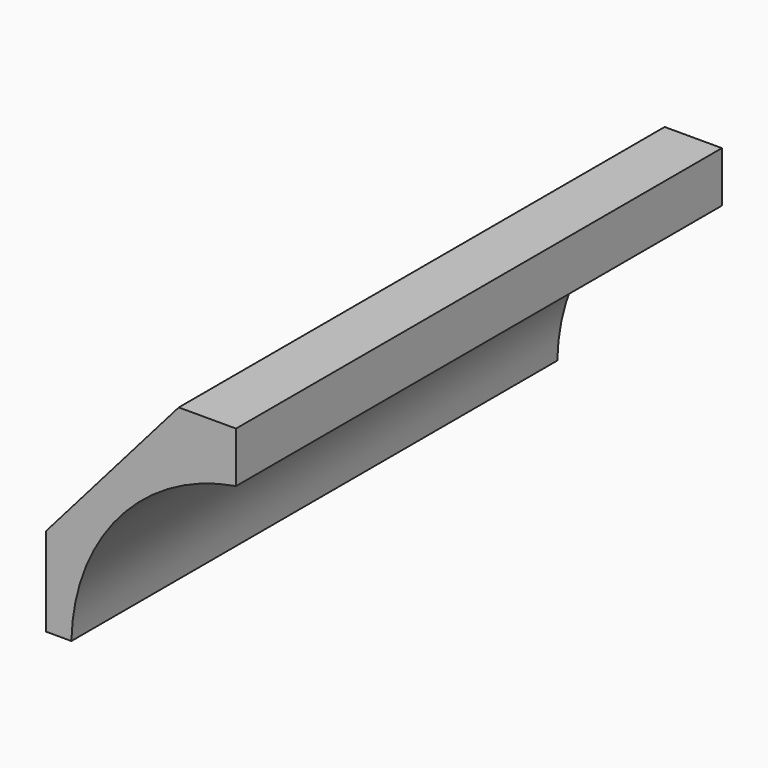
from build123d import *

# Parameters (mm, degrees)
F1_DEPTH = 152.4


# Not quite as in the source:
# - ends of sketch curves that miss each other by under 0.0002 mm in the source are joined


with BuildPart() as f1:
    # F0 (on Front) → F1 (new body)
    with BuildSketch(Plane.XZ):
        with BuildLine():
            Line((23.8291116, 17.474692), (23.8291116, 30.1835566))
            Line((23.8291116, 30.1835566), (9.4594934, 30.1835566))
            Line((9.4594934, 30.1835566), (-23.8291116, -7.9430372))
            Line((-23.8291116, -7.9430372), (-23.8291116, -30.1835566))
            Line((-23.8291116, -30.1835566), (-17.474692, -30.1835566))
            ThreePointArc((-17.474692, -30.1835566), (-5.4486786774, 1.121334901), (23.8291116, 17.474692))
        make_face()
    extrude(amount=F1_DEPTH)


solid = f1.part
